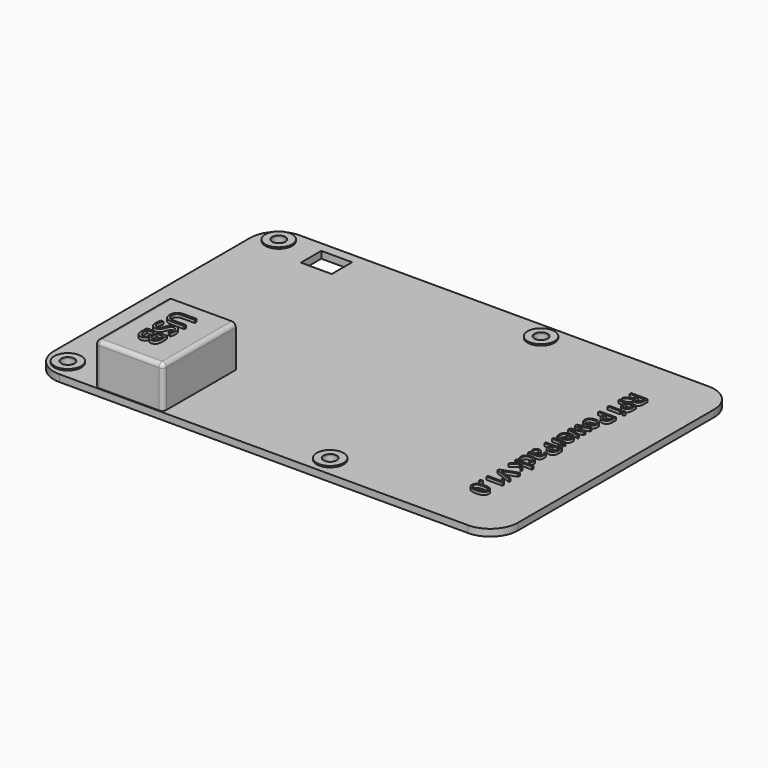
from build123d import *

# Parameters (mm, degrees)
F0_W           = 85.09
F0_H           = 55.118
F1_DEPTH       = 1.27
F2_R           = 5.08
F3_R           = 1.2109116799
F4_DEPTH       = 1.27
F5_W           = 63.5
F5_H           = 38.1
F6_DEPTH       = 6.35
F7_F1_R        = 5.08
F7_F2_R        = 5.08
F7_F3_R        = 5.08
F7_F4_R        = 5.08
F9_W           = 5.6576728821
F9_H           = 4.6750153415
F10_DEPTH      = 5.08
F11_W          = 12.4787762761
F11_H          = 16.6547195404
F12_DEPTH      = 7.62
F13_TEXT_SIZE  = 4.1753424658
F14_DEPTH      = 0.508
F15_R          = 0.762
F16_TEXT_SIZE  = 5.2519182619
F17_DEPTH      = 0.508
F3_R_2         = 2.4693873006
F18_DEPTH      = 0.254
F18_DEPTH_BACK = 1.524


# Not quite as in the source:
# - a feature of the source that left no trace in its solid (it failed there, or was rolled back) is left out
# - Text() gives the source's letters only with a copy of the font that has no kerning and outlines rounded to 1/6400 em; it was checked with that copy


with BuildPart() as f1:
    # F0 (on Top) → F1 (new body)
    with BuildSketch(Plane.XY):
        with Locations((42.545, -27.559)):
            Rectangle(F0_W, F0_H)
    extrude(amount=F1_DEPTH)

    # F2
    f2_edges = [f1.edges().sort_by_distance(p)[0] for p in [
        (85.09, -55.118, 0.635),
        (0, -55.118, 0.635),
        (85.09, 0, 0.635),
        (0, 0, 0.635),
    ]]
    fillet(f2_edges, radius=F2_R)

    # F3 (on face) → F4 (cut)
    with BuildSketch(Plane.XY.offset(1.27)):
        with Locations((51.8668480217, -3.2243323512)):
            Circle(F3_R)
        with Locations((51.8668480217, -51.5464544296)):
            Circle(F3_R)
        with Locations((3.7787982728, -3.2243323512)):
            Circle(F3_R)
        with Locations((3.7787982728, -51.5464544296)):
            Circle(F3_R)
    extrude(amount=-F4_DEPTH, mode=Mode.SUBTRACT)

    # F5 (on face) → F6 (join)
    with BuildSketch(Plane(origin=(0, 0, 0), x_dir=(1, 0, 0), z_dir=(0, 0, -1))):
        with Locations((34.2887183125, 27.6673909605)):
            Rectangle(F5_W, F5_H)
    extrude(amount=F6_DEPTH)

    # F7: fillet of radius 5.08 on 4 edges, made by hand

    # F7_f1
    f7_f1_edges = [f1.edges().sort_by_distance(p)[0] for p in [
        (2.5387183125, -27.6673909605, -6.35),
    ]]
    fillet(f7_f1_edges, radius=F7_F1_R)

    # F7_f2
    f7_f2_edges = [f1.edges().sort_by_distance(p)[0] for p in [
        (36.8287183125, -46.7173909605, -6.35),
    ]]
    fillet(f7_f2_edges, radius=F7_F2_R)

    # F7_f3
    f7_f3_edges = [f1.edges().sort_by_distance(p)[0] for p in [
        (66.0387183125, -25.1273909605, -6.35),
    ]]
    fillet(f7_f3_edges, radius=F7_F3_R)

    # F7_f4
    f7_f4_edges = [f1.edges().sort_by_distance(p)[0] for p in [
        (34.2887183125, -8.6173909605, -6.35),
    ]]
    fillet(f7_f4_edges, radius=F7_F4_R)

    # F9 (on face) → F10 (cut)
    with BuildSketch(Plane.XY.offset(1.27)):
        with Locations((13.2903270423, -4.1677228874)):
            Rectangle(F9_W, F9_H)
    extrude(amount=-F10_DEPTH, mode=Mode.SUBTRACT)

    # F11 (on face) → F12 (join)
    with BuildSketch(Plane.XY.offset(1.27)):
        with Locations((17.7275864407, -46.6259601817)):
            Rectangle(F11_W, F11_H)
    extrude(amount=F12_DEPTH)

    # F13 (on face) → F14 (join)
    with BuildSketch(Plane.XY.offset(1.27)):
        with Locations(Location((73.2543265125, -8.8890084725), (0, 0, -90))):
            Text('RPi PowerPack V1.0', F13_TEXT_SIZE, font='Open Sans', text_align=(TextAlign.LEFT, TextAlign.BOTTOM))
    extrude(amount=F14_DEPTH)

    # F15
    f15_edges = [f1.edges().sort_by_distance(p)[0] for p in [
        (11.488198, -46.62596, 8.89),
        (23.966975, -46.62596, 8.89),
        (17.727586, -54.95332, 8.89),
        (23.966975, -54.95332, 5.08),
        (11.488198, -54.95332, 5.08),
    ]]
    fillet(f15_edges, radius=F15_R)

    # F16 (on face) → F17 (join)
    with BuildSketch(Plane.XY.offset(8.89)):
        with Locations(Location((15.7034727366, -41.1436107057), (0, 0, -90))):
            Text('USB', F16_TEXT_SIZE, font='Open Sans', text_align=(TextAlign.LEFT, TextAlign.BOTTOM))
    extrude(amount=F17_DEPTH)

    # F3 (on face) → F18 (join, two sides)
    with BuildSketch(Plane.XY.offset(1.27)) as f18_sk:
        with Locations((51.8668480217, -3.2243323512)):
            Circle(F3_R_2)
        with Locations((51.8668480217, -3.2243323512)):
            Circle(F3_R, mode=Mode.SUBTRACT)
        with Locations((51.8668480217, -51.5464544296)):
            Circle(F3_R_2)
        with Locations((51.8668480217, -51.5464544296)):
            Circle(F3_R, mode=Mode.SUBTRACT)
        with Locations((3.7787982728, -3.2243323512)):
            Circle(F3_R_2)
        with Locations((3.7787982728, -3.2243323512)):
            Circle(F3_R, mode=Mode.SUBTRACT)
        with Locations((3.7787982728, -51.5464544296)):
            Circle(F3_R_2)
        with Locations((3.7787982728, -51.5464544296)):
            Circle(F3_R, mode=Mode.SUBTRACT)
    extrude(amount=F18_DEPTH)
    extrude(f18_sk.sketch, amount=-F18_DEPTH_BACK)


solid = f1.part
